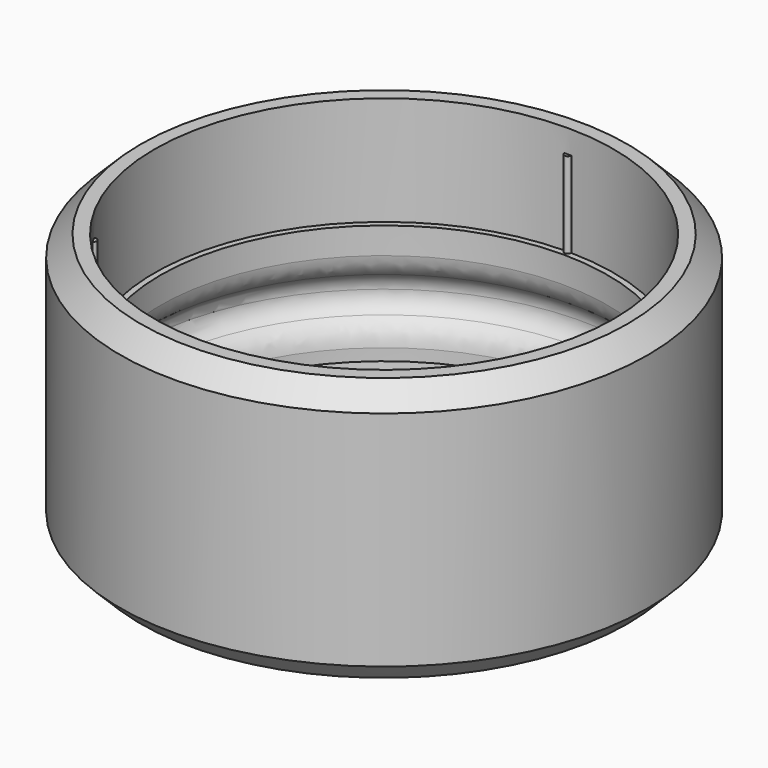
from build123d import *

# Parameters (mm, degrees)
F2_SIZE  = 1.2
F3_R     = 1.6
F5_DEPTH = 5


# Not quite as in the source:
# - a feature names something its author has since deleted; it is built from what else it names


with BuildPart() as f1:
    # F0 (on Front) → F1 (revolve)
    with BuildSketch(Plane.XZ):
        with BuildLine():
            ThreePointArc((13.05, 6.2909673646), (14.0291561976, 5.9854143467), (14.45, 5.05))
            ThreePointArc((14.45, 5.05), (14.0838834765, 4.1661165235), (13.2, 3.8))
            Line((13.2, 3.8), (13.2, 2))
            Line((13.2, 2), (11, 2))
            Line((11, 2), (11, 0))
            Line((11, 0), (15.4, 0))
            Line((15.4, 0), (15.4, 15.4))
            Line((15.4, 15.4), (13.4, 15.4))
            Line((13.4, 15.4), (13.4, 9.05))
            Line((13.4, 9.05), (13.05, 9.05))
            Line((13.05, 9.05), (13.05, 6.2909673646))
        make_face()
    revolve(axis=Axis((0, 0, 9.4043305144), (0, 0, 1)))

    # F2
    f2_edges = [f1.edges().sort_by_distance(p)[0] for p in [
        (-11, 0, 0),
        (-15.4, 0, 0),
        (-15.4, 0, 15.4),
    ]]
    chamfer(f2_edges, length=F2_SIZE)

    # F3
    f3_edges = [f1.edges().sort_by_distance(p)[0] for p in [
        (-13.05, 0, 6.290967),
        (-13.2, 0, 3.8),
    ]]
    fillet(f3_edges, radius=F3_R)

    # F4 (on face) → F5 (join)
    with BuildSketch(Plane.XY.offset(9.05)):
        with BuildLine():
            ThreePointArc((0.1999944308, 13.3985074627), (0.1999986077, 13.3992537261), (0.2, 13.4))
            ThreePointArc((0.2, 13.4), (-0.0007462739, 13.5999986077), (-0.1999944308, 13.3985074627))
            ThreePointArc((-0.1999944308, 13.3985074627), (0, 13.4), (0.1999944308, 13.3985074627))
        make_face()
        with BuildLine():
            ThreePointArc((0.1999944308, 13.3985074627), (0, 13.4), (-0.1999944308, 13.3985074627))
            ThreePointArc((-0.1999944308, 13.3985074627), (0, 13.2), (0.1999944308, 13.3985074627))
        make_face()
        with BuildLine():
            ThreePointArc((-11.4047404107, -6.7), (-11.5040948148, -6.527169262), (-11.7034450509, -6.5260534737))
            ThreePointArc((-11.7034450509, -6.5260534737), (-11.6047404107, -6.7), (-11.5034506201, -6.872453989))
            ThreePointArc((-11.5034506201, -6.872453989), (-11.4311633988, -6.7993530117), (-11.4047404107, -6.7))
        make_face()
        with BuildLine():
            ThreePointArc((11.5034506201, -6.872453989), (11.6047404107, -6.7), (11.7034450509, -6.5260534737))
            ThreePointArc((11.7034450509, -6.5260534737), (11.43153533, -6.6), (11.5034506201, -6.872453989))
        make_face()
    extrude(amount=F5_DEPTH)


solid = f1.part
